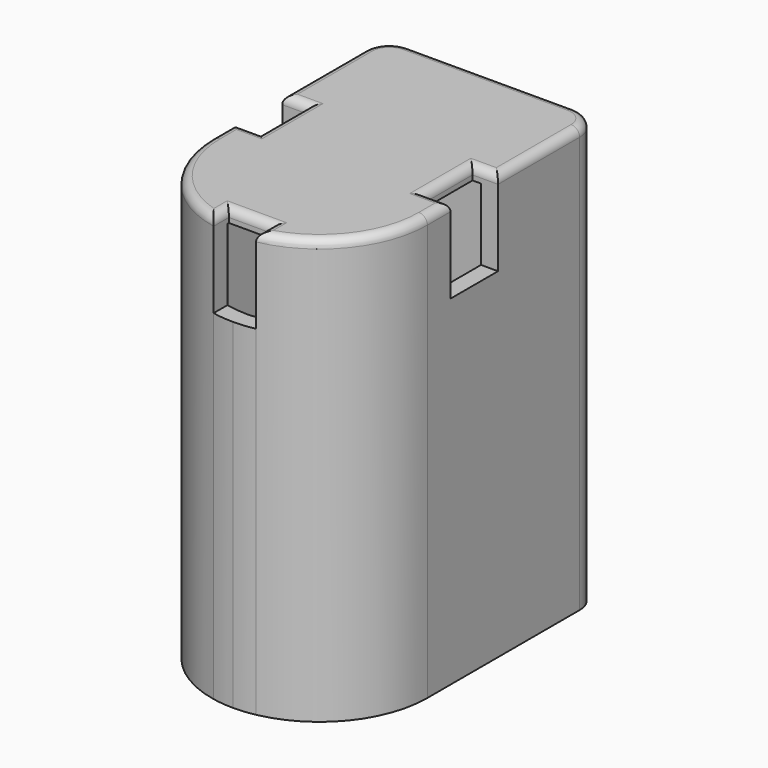
from build123d import *
from build123d import SkipClean  # not in build123d's __all__

# Parameters (mm, degrees)
F1_DEPTH = 10
F0_W     = 3
F0_H     = 7
F2_DEPTH = 40
F4_DEPTH = 48.42995
F5_R     = 1


# Not quite as in the source:
# - after a boolean that leaves OpenCascade's solid faulty, fix() repairs it


with BuildPart() as f1:
    # F0 (on Top) → F1 (new body)
    with BuildSketch(Plane.XY):
        with BuildLine():
            ThreePointArc((12.7, 16.05), (11.8213203436, 18.1713203436), (9.7, 19.05))
            Line((9.7, 19.05), (-9.7, 19.05))
            ThreePointArc((-9.7, 19.05), (-11.8213203436, 18.1713203436), (-12.7, 16.05))
            Line((-12.7, 16.05), (-12.7, 4.05))
            Line((-12.7, 4.05), (-9.7, 4.05))
            Line((-9.7, 4.05), (-9.7, -2.95))
            Line((-9.7, -2.95), (-12.7, -2.95))
            Line((-12.7, -2.95), (-12.7, -6.35))
            ThreePointArc((-12.7, -6.35), (-9.8244592727, -14.3979811133), (-2.5, -18.801505933))
            Line((-2.5, -18.801505933), (-2.5, -16.55))
            Line((-2.5, -16.55), (2.5, -16.55))
            Line((2.5, -16.55), (2.5, -18.801505933))
            ThreePointArc((2.5, -18.801505933), (9.8244592727, -14.3979811133), (12.7, -6.35))
            Line((12.7, -6.35), (12.7, -2.95))
            Line((12.7, -2.95), (9.7, -2.95))
            Line((9.7, -2.95), (9.7, 4.05))
            Line((9.7, 4.05), (12.7, 4.05))
            Line((12.7, 4.05), (12.7, 16.05))
        make_face()
    extrude(amount=F1_DEPTH)

    # F0 (on Top) → F2 (join)
    with BuildSketch(Plane.XY):
        with BuildLine():
            ThreePointArc((12.7, 16.05), (11.8213203436, 18.1713203436), (9.7, 19.05))
            Line((9.7, 19.05), (-9.7, 19.05))
            ThreePointArc((-9.7, 19.05), (-11.8213203436, 18.1713203436), (-12.7, 16.05))
            Line((-12.7, 16.05), (-12.7, 4.05))
            Line((-12.7, 4.05), (-9.7, 4.05))
            Line((-9.7, 4.05), (-9.7, -2.95))
            Line((-9.7, -2.95), (-12.7, -2.95))
            Line((-12.7, -2.95), (-12.7, -6.35))
            ThreePointArc((-12.7, -6.35), (-9.8244592727, -14.3979811133), (-2.5, -18.801505933))
            Line((-2.5, -18.801505933), (-2.5, -16.55))
            Line((-2.5, -16.55), (2.5, -16.55))
            Line((2.5, -16.55), (2.5, -18.801505933))
            ThreePointArc((2.5, -18.801505933), (9.8244592727, -14.3979811133), (12.7, -6.35))
            Line((12.7, -6.35), (12.7, -2.95))
            Line((12.7, -2.95), (9.7, -2.95))
            Line((9.7, -2.95), (9.7, 4.05))
            Line((9.7, 4.05), (12.7, 4.05))
            Line((12.7, 4.05), (12.7, 16.05))
        make_face()
        with Locations((11.2, 0.55)):
            Rectangle(F0_W, F0_H)
        with BuildLine():
            ThreePointArc((0, -19.05), (1.2561597531, -18.9877237933), (2.5, -18.801505933))
            Line((2.5, -18.801505933), (2.5, -16.55))
            Line((2.5, -16.55), (-2.5, -16.55))
            Line((-2.5, -16.55), (-2.5, -18.801505933))
            ThreePointArc((-2.5, -18.801505933), (-1.2561597531, -18.9877237933), (0, -19.05))
        make_face()
        with Locations((-11.2, 0.55)):
            Rectangle(F0_W, F0_H)
    with SkipClean():  # cleaning this boolean's faces spoils the solid; the shape is the same uncleaned
        extrude(amount=-F2_DEPTH)

    # F3 (on face) → F4 (cut)
    with BuildSketch(Plane(origin=(0, 0, -40), x_dir=(1, 0, 0), z_dir=(0, 0, -1))):
        with BuildLine():
            ThreePointArc((10.7, 6.35), (0, 17.05), (-10.7, 6.35))
            Line((-10.7, 6.35), (-10.7, -17.05))
            Line((-10.7, -17.05), (10.7, -17.05))
            Line((10.7, -17.05), (10.7, 6.35))
        make_face()
    extrude(amount=-F4_DEPTH, mode=Mode.SUBTRACT)

    add(f1.part.fix(), mode=Mode.REPLACE)

    # F5
    f5_edges = [f1.edges().sort_by_distance(p)[0] for p in [
        (9.824459, -14.397981, 10),
        (12.7, -4.65, 10),
        (11.2, -2.95, 10),
        (9.7, 0.55, 10),
        (11.2, 4.05, 10),
        (12.7, 10.05, 10),
        (11.82132, 18.17132, 10),
        (0, 19.05, 10),
        (-11.82132, 18.17132, 10),
        (-12.7, 10.05, 10),
        (-11.2, 4.05, 10),
        (-9.7, 0.55, 10),
        (-11.2, -2.95, 10),
        (-12.7, -4.65, 10),
        (-9.824459, -14.397981, 10),
        (-2.5, -17.675753, 10),
        (0, -16.55, 10),
        (2.5, -17.675753, 10),
    ]]
    fillet(f5_edges, radius=F5_R)


solid = f1.part
